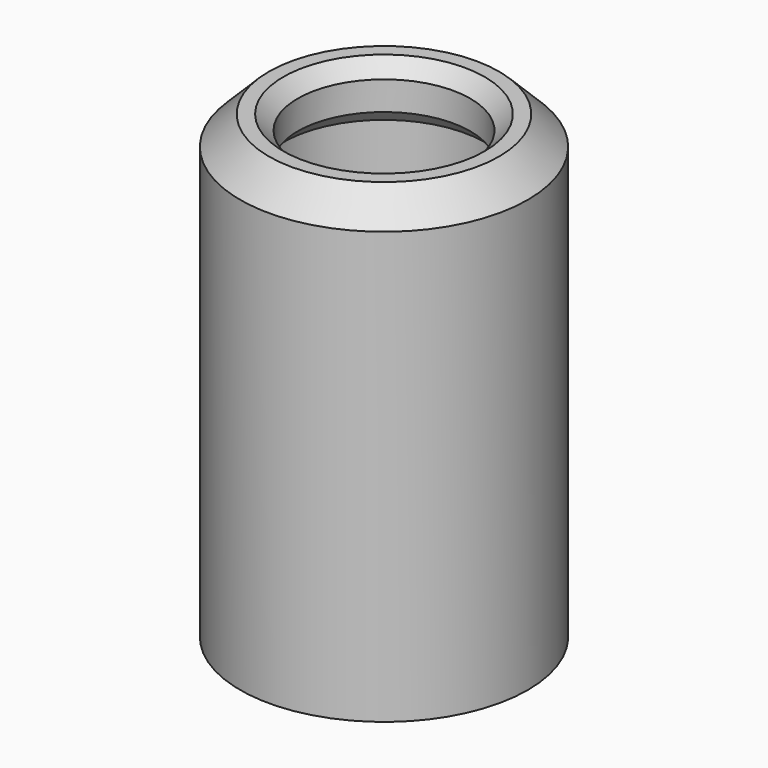
from build123d import *

# Parameters (mm, degrees)
F0_R     = 7.9375
F0_R_2   = 4.7625
F1_DEPTH = 25.4
F2_SIZE  = 1.5875
F3_W     = 5.55625
F3_H     = 19.05
F5_SIZE  = 0.79374


# Not quite as in the source:
# - a fillet or chamfer is up to 0.001 mm smaller than in the source, because OpenCascade refuses the exact size


with BuildPart() as f1:
    # F0 (on Top) → F1 (new body)
    with BuildSketch(Plane.XY):
        Circle(F0_R)
        Circle(F0_R_2, mode=Mode.SUBTRACT)
    extrude(amount=F1_DEPTH)

    # F2
    f2_edges = [f1.edges().sort_by_distance(p)[0] for p in [
        (-7.9375, 0, 25.4),
    ]]
    chamfer(f2_edges, length=F2_SIZE)

    # F3 (on Front) → F4 (revolve, cut)
    with BuildSketch(Plane.XZ):
        with Locations((2.778125, 12.7)):
            Rectangle(F3_W, F3_H)
    revolve(axis=Axis((0, 0, 0), (0, 0, -1)), mode=Mode.SUBTRACT)

    # F5 (size 0.79375 in the source; OpenCascade refuses exactly that, so slightly less here)
    f5_edges = [f1.edges().sort_by_distance(p)[0] for p in [
        (-4.7625, 0, 0),
        (-4.7625, 0, 3.175),
        (-4.7625, 0, 22.225),
        (-4.7625, 0, 25.4),
    ]]
    chamfer(f5_edges, length=F5_SIZE)


solid = f1.part
